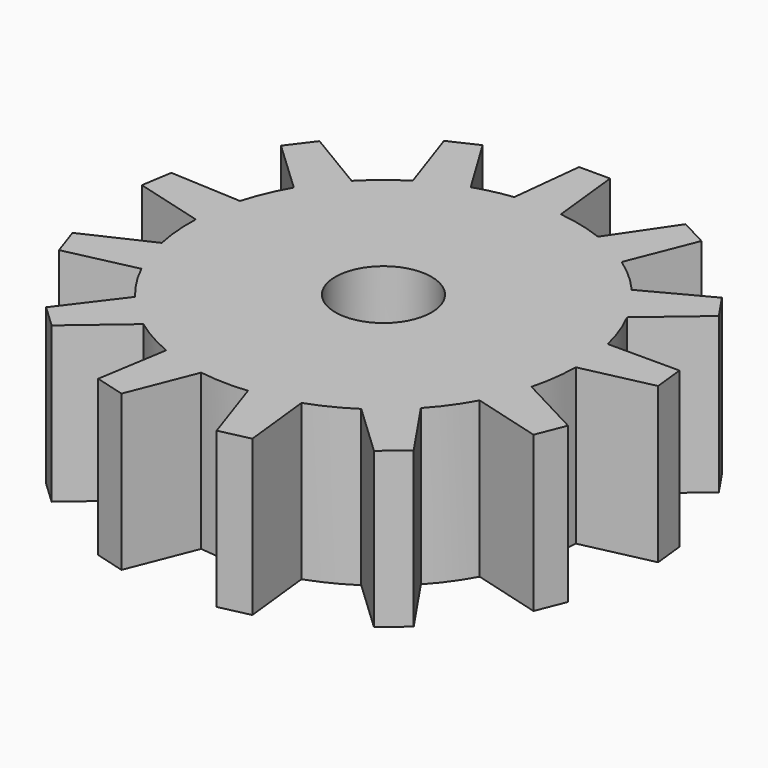
from build123d import *

# Parameters (mm, degrees)
F0_R     = 3.1
F1_DEPTH = 10


# Not quite as in the source:
# - a feature names something its author has since deleted; it is built from what else it names


with BuildPart() as f1:
    # F0 (on Top) → F1 (new body)
    with BuildSketch(Plane.XY):
        with BuildLine():
            Line((11.7831534795, -12.2946042669), (9.1877297548, -8.4755897702))
            ThreePointArc((9.1877297548, -8.4755897702), (8.1042674519, -9.516871811), (6.9036805201, -10.4206139587))
            Line((6.9036805201, -10.4206139587), (10.2604539897, -13.5912870592))
            Line((10.2604539897, -13.5912870592), (11.7831534795, -12.2946042669))
        make_face()
        with BuildLine():
            ThreePointArc((9.4254531567, 8.2104100258), (10.3425930143, 7.0200263348), (11.110259477, 5.7281877024))
            Line((11.110259477, 5.7281877024), (14.6275286062, 8.7198283742))
            Line((14.6275286062, 8.7198283742), (13.5043243926, 10.3746432565))
            Line((13.5043243926, 10.3746432565), (9.4254531567, 8.2104100258))
        make_face()
        with BuildLine():
            Line((16.1681140592, -5.3471569801), (12.0867087003, -3.1877065099))
            ThreePointArc((12.0867087003, -3.1877065099), (11.6168440528, -4.6150768414), (10.9790902584, -5.9757490826))
            Line((10.9790902584, -5.9757490826), (15.4297017645, -7.2058520285))
            Line((15.4297017645, -7.2058520285), (16.1681140592, -5.3471569801))
        make_face()
        with BuildLine():
            ThreePointArc((-6.6040163856, 10.6130564673), (-5.2827282718, 11.328847338), (-3.8850930245, 11.8809112526))
            Line((-3.8850930245, 11.8809112526), (-6.2782026626, 15.8298506414))
            Line((-6.2782026626, 15.8298506414), (-8.0908182366, 14.9846141179))
            Line((-8.0908182366, 14.9846141179), (-6.6040163856, 10.6130564673))
        make_face()
        with BuildLine():
            Line((-10.9387342022, -13.0515935446), (-7.4249743059, -10.0558319674))
            ThreePointArc((-7.4249743059, -10.0558319674), (-8.5780204734, -9.0921705197), (-9.6070952306, -7.9971070538))
            Line((-9.6070952306, -7.9971070538), (-12.3934814853, -11.6791102689))
            Line((-12.3934814853, -11.6791102689), (-10.9387342022, -13.0515935446))
        make_face()
        with BuildLine():
            ThreePointArc((4.484602064, 11.6678337461), (5.8523358933, 11.0453684679), (7.1354904963, 10.2632731318))
            Line((7.1354904963, 10.2632731318), (8.8428062923, 14.5535142449))
            Line((8.8428062923, 14.5535142449), (7.0755473374, 15.4898879879))
            Line((7.0755473374, 15.4898879879), (4.484602064, 11.6678337461))
        make_face()
        with BuildLine():
            ThreePointArc((-10.8043972519, 6.2860957696), (-9.9719920146, 7.5371994308), (-8.9954693884, 8.6793738531))
            Line((-8.9954693884, 8.6793738531), (-12.9589331854, 11.0483505871))
            Line((-12.9589331854, 11.0483505871), (-14.1648850944, 9.4528318648))
            Line((-14.1648850944, 9.4528318648), (-10.8043972519, 6.2860957696))
        make_face()
        with BuildLine():
            Line((-3.5552032377, -16.6541445274), (-1.8529176571, -12.3619050375))
            ThreePointArc((-1.8529176571, -12.3619050375), (-3.3229568779, -12.0502264538), (-4.744972006, -11.5643953868))
            Line((-4.744972006, -11.5643953868), (-5.4832394703, -16.1224714269))
            Line((-5.4832394703, -16.1224714269), (-3.5552032377, -16.6541445274))
        make_face()
        with BuildLine():
            ThreePointArc((-12.4901514097, 0.4961025726), (-12.340363914, 1.9913358508), (-12.0122308055, 3.457789912))
            Line((-12.0122308055, 3.457789912), (-16.6235880549, 3.6954458703))
            Line((-16.6235880549, 3.6954458703), (-16.9422017911, 1.720987644))
            Line((-16.9422017911, 1.720987644), (-12.4901514097, 0.4961025726))
        make_face()
        with BuildLine():
            Line((-15.7763727361, -6.4114010396), (-11.2689346746, -5.4093540556))
            ThreePointArc((-11.2689346746, -5.4093540556), (-11.8366266187, -4.0179933163), (-12.2332530705, -2.5685636671))
            Line((-12.2332530705, -2.5685636671), (-16.4192516667, -4.5175407807))
            Line((-16.4192516667, -4.5175407807), (-15.7763727361, -6.4114010396))
        make_face()
        with BuildLine():
            ThreePointArc((12.1726144308, 2.8420868951), (12.4178838854, 1.4304404243), (12.5, 0))
            ThreePointArc((12.5, 0), (12.4998037623, -0.0700421594), (12.4992150553, -0.1400821196))
            Line((12.4992150553, -0.1400821196), (17.0078246246, 0.8566805343))
            Line((17.0078246246, 0.8566805343), (16.7900908749, 2.8447932107))
            Line((16.7900908749, 2.8447932107), (12.1726144308, 2.8420868951))
        make_face()
        with BuildLine():
            Line((4.6557694441, -16.3805925071), (4.1503889837, -11.7908554093))
            ThreePointArc((4.1503889837, -11.7908554093), (2.7054951742, -12.203700089), (1.2215009624, -12.4401742511))
            Line((1.2215009624, -12.4401742511), (2.7031774298, -16.813471735))
            Line((2.7031774298, -16.813471735), (4.6557694441, -16.3805925071))
        make_face()
        with BuildLine():
            ThreePointArc((-1.5, 12.409673646), (0, 12.5), (1.5, 12.409673646))
            Line((1.5, 12.409673646), (1, 17))
            Line((1, 17), (-1, 17))
            Line((-1, 17), (-1.5, 12.409673646))
        make_face()
        with BuildLine():
            ThreePointArc((-4.744972006, -11.5643953868), (-3.3229568779, -12.0502264538), (-1.8529176571, -12.3619050375))
            Line((-1.8529176571, -12.3619050375), (-4.744972006, -11.5643953868))
        make_face()
        with BuildLine():
            Line((4.484602064, 11.6678337461), (7.1354904963, 10.2632731318))
            ThreePointArc((7.1354904963, 10.2632731318), (5.8523358933, 11.0453684679), (4.484602064, 11.6678337461))
        make_face()
        with BuildLine():
            Line((-10.8043972519, 6.2860957696), (-8.9954693884, 8.6793738531))
            ThreePointArc((-8.9954693884, 8.6793738531), (-9.9719920146, 7.5371994308), (-10.8043972519, 6.2860957696))
        make_face()
        with BuildLine():
            ThreePointArc((-12.2332530705, -2.5685636671), (-11.8366266187, -4.0179933163), (-11.2689346746, -5.4093540556))
            Line((-11.2689346746, -5.4093540556), (-12.2332530705, -2.5685636671))
        make_face()
        with BuildLine():
            ThreePointArc((10.9790902584, -5.9757490826), (11.6168440528, -4.6150768414), (12.0867087003, -3.1877065099))
            Line((12.0867087003, -3.1877065099), (10.9790902584, -5.9757490826))
        make_face()
        with BuildLine():
            Line((-12.4901514097, 0.4961025726), (-12.0122308055, 3.457789912))
            ThreePointArc((-12.0122308055, 3.457789912), (-12.340363914, 1.9913358508), (-12.4901514097, 0.4961025726))
        make_face()
        with BuildLine():
            ThreePointArc((-9.6070952306, -7.9971070538), (-8.5780204734, -9.0921705197), (-7.4249743059, -10.0558319674))
            Line((-7.4249743059, -10.0558319674), (-9.6070952306, -7.9971070538))
        make_face()
        with BuildLine():
            ThreePointArc((12.4992150553, -0.1400821196), (12.4998037623, -0.0700421594), (12.5, 0))
            ThreePointArc((12.5, 0), (12.4178838854, 1.4304404243), (12.1726144308, 2.8420868951))
            Line((12.1726144308, 2.8420868951), (12.4992150553, -0.1400821196))
        make_face()
        with BuildLine():
            Line((-6.6040163856, 10.6130564673), (-3.8850930245, 11.8809112526))
            ThreePointArc((-3.8850930245, 11.8809112526), (-5.2827282718, 11.328847338), (-6.6040163856, 10.6130564673))
        make_face()
        with BuildLine():
            ThreePointArc((1.2215009624, -12.4401742511), (2.7054951742, -12.203700089), (4.1503889837, -11.7908554093))
            Line((4.1503889837, -11.7908554093), (1.2215009624, -12.4401742511))
        make_face()
        with BuildLine():
            Line((9.4254531567, 8.2104100258), (11.110259477, 5.7281877024))
            ThreePointArc((11.110259477, 5.7281877024), (10.3425930143, 7.0200263348), (9.4254531567, 8.2104100258))
        make_face()
        with BuildLine():
            ThreePointArc((6.9036805201, -10.4206139587), (8.1042674519, -9.516871811), (9.1877297548, -8.4755897702))
            Line((9.1877297548, -8.4755897702), (6.9036805201, -10.4206139587))
        make_face()
        with BuildLine():
            Line((-1.5, 12.409673646), (1.5, 12.409673646))
            ThreePointArc((1.5, 12.409673646), (0, 12.5), (-1.5, 12.409673646))
        make_face()
        with BuildLine():
            Line((12.4992150553, -0.1400821196), (12.1726144308, 2.8420868951))
            ThreePointArc((12.1726144308, 2.8420868951), (11.7305348906, 4.3179336703), (11.110259477, 5.7281877024))
            Line((11.110259477, 5.7281877024), (9.4254531567, 8.2104100258))
            ThreePointArc((9.4254531567, 8.2104100258), (8.3438465591, 9.3075359037), (7.1354904963, 10.2632731318))
            Line((7.1354904963, 10.2632731318), (4.484602064, 11.6678337461))
            ThreePointArc((4.484602064, 11.6678337461), (3.0152026591, 12.1308925032), (1.5, 12.409673646))
            Line((1.5, 12.409673646), (-1.5, 12.409673646))
            ThreePointArc((-1.5, 12.409673646), (-2.7054951742, 12.203700089), (-3.8850930245, 11.8809112526))
            Line((-3.8850930245, 11.8809112526), (-6.6040163856, 10.6130564673))
            ThreePointArc((-6.6040163856, 10.6130564673), (-7.8594383525, 9.7200426328), (-8.9954693884, 8.6793738531))
            Line((-8.9954693884, 8.6793738531), (-10.8043972519, 6.2860957696))
            ThreePointArc((-10.8043972519, 6.2860957696), (-11.4956277551, 4.9092303386), (-12.0122308055, 3.457789912))
            Line((-12.0122308055, 3.457789912), (-12.4901514097, 0.4961025726))
            ThreePointArc((-12.4901514097, 0.4961025726), (-12.4563127395, -1.0441613555), (-12.2332530705, -2.5685636671))
            Line((-12.2332530705, -2.5685636671), (-11.2689346746, -5.4093540556))
            ThreePointArc((-11.2689346746, -5.4093540556), (-10.5179024784, -6.7545338443), (-9.6070952306, -7.9971070538))
            Line((-9.6070952306, -7.9971070538), (-7.4249743059, -10.0558319674))
            ThreePointArc((-7.4249743059, -10.0558319674), (-6.131544602, -10.8928490669), (-4.744972006, -11.5643953868))
            Line((-4.744972006, -11.5643953868), (-1.8529176571, -12.3619050375))
            ThreePointArc((-1.8529176571, -12.3619050375), (-0.3181246266, -12.4959512132), (1.2215009624, -12.4401742511))
            Line((1.2215009624, -12.4401742511), (4.1503889837, -11.7908554093))
            ThreePointArc((4.1503889837, -11.7908554093), (5.5693360069, -11.1907326142), (6.9036805201, -10.4206139587))
            Line((6.9036805201, -10.4206139587), (9.1877297548, -8.4755897702))
            ThreePointArc((9.1877297548, -8.4755897702), (10.1605835574, -7.2809712108), (10.9790902584, -5.9757490826))
            Line((10.9790902584, -5.9757490826), (12.0867087003, -3.1877065099))
            ThreePointArc((12.0867087003, -3.1877065099), (12.3870462717, -1.6766289583), (12.4992150553, -0.1400821196))
        make_face()
        Circle(F0_R, mode=Mode.SUBTRACT)
    extrude(amount=F1_DEPTH)


solid = f1.part
